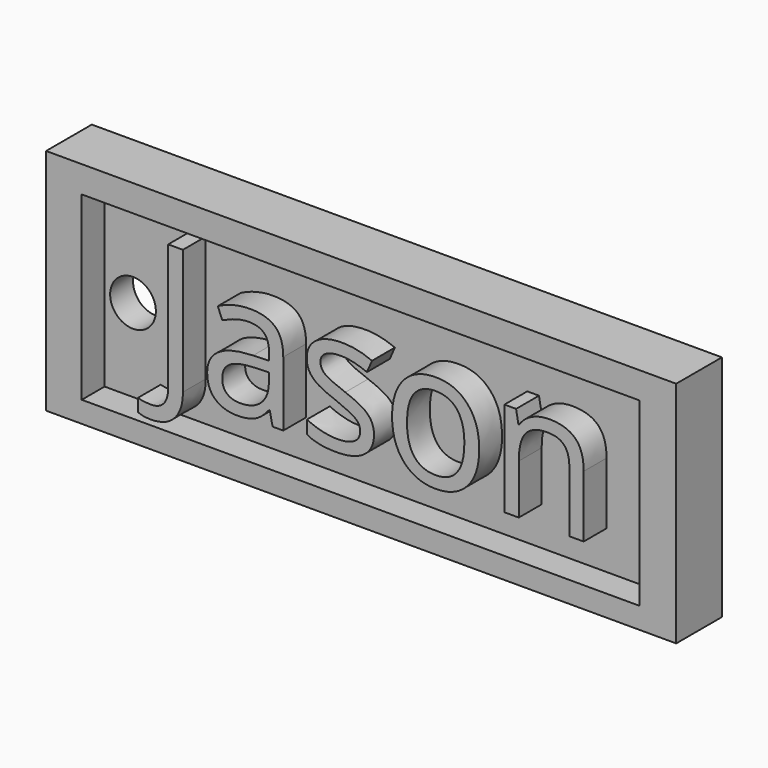
from build123d import *

# Parameters (mm, degrees)
F0_W         = 70
F0_H         = 25.4
F0_W_2       = 61.9557951577
F0_H_2       = 20.0872323476
F1_DEPTH     = 6.35
F2_DEPTH     = 3.175
F3_R         = 2.54
F4_DEPTH     = 25.4
F5_TEXT_SIZE = 19.6863457463
F6_DEPTH     = 3.175


# Not quite as in the source:
# - Text() gives the source's letters only with a copy of the font that has no kerning and outlines rounded to 1/6400 em; it was checked with that copy


with BuildPart() as f1:
    # F0 (on Front) → F1 (new body)
    with BuildSketch(Plane.XZ):
        with Locations((35, 12.7)):
            Rectangle(F0_W, F0_H)
        with Locations((34.9397433456, 12.3975903261)):
            Rectangle(F0_W_2, F0_H_2, mode=Mode.SUBTRACT)
    extrude(amount=F1_DEPTH)

    # F0 (on Front) → F2 (join)
    with BuildSketch(Plane.XZ):
        with Locations((34.9397433456, 12.3975903261)):
            Rectangle(F0_W_2, F0_H_2)
    extrude(amount=F2_DEPTH)

    # F3 (on face) → F4 (cut)
    with BuildSketch(Plane.XZ.offset(3.175)):
        with Locations((7.1169661364, 11.5709906414)):
            Circle(F3_R)
    extrude(amount=-F4_DEPTH, mode=Mode.SUBTRACT)

    # F5 (on face) → F6 (join)
    with BuildSketch(Plane.XZ.offset(3.175)):
        with Locations((11.7374188078, 6.6215020605)):
            Text('Jason', F5_TEXT_SIZE, font='Open Sans', text_align=(TextAlign.LEFT, TextAlign.BOTTOM))
    extrude(amount=F6_DEPTH)


solid = f1.part
